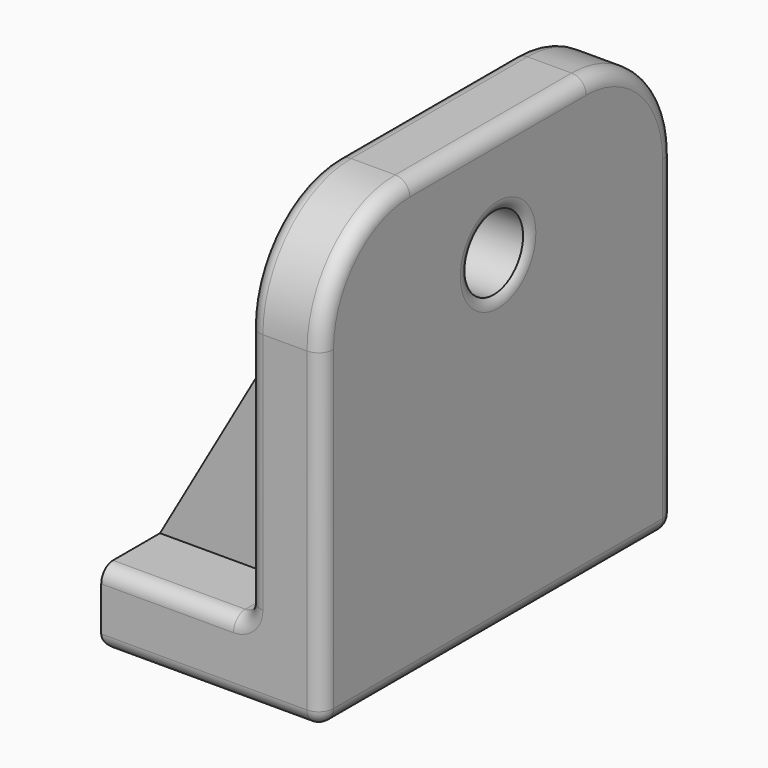
from build123d import *

# Parameters (mm, degrees)
F1_DEPTH  = 76.2
F2_R      = 12.7
F3_DEPTH  = 76.201
F5_DEPTH  = 25.401
F6_R      = 38.1
F7_R      = 38.1
F10_DEPTH = 6.35
F11_SIZE  = 1.524
F12_SIZE  = 1.524
F13_R     = 5.08


# Not quite as in the source:
# - a length typed as a fraction of an inch, garbled in the dataset ("3 / 203.2 mm" for 3/8 in), is restored
# - a pattern or mirror of a feature is missing from the dataset's text; its kind, count and spacing are read off the source's solid


with BuildPart() as f1:
    # F0 (on Front) → F1 (new body, symmetric)
    with BuildSketch(Plane.XZ):
        Polygon((-76.2, 0), (0, 0), (0, 152.4), (-25.4, 152.4), (-25.4, 25.4), (-76.2, 25.4), align=None)
    extrude(amount=F1_DEPTH, both=True)

    # F2 (on face) → F3 (cut, through all)
    with BuildSketch(Plane.YZ):
        with Locations((0, 114.3)):
            Circle(F2_R)
    extrude(amount=-F3_DEPTH, mode=Mode.SUBTRACT)

    # F4 (on face) → F5 (cut, through all)
    with BuildSketch(Plane.XY.offset(25.4)):
        with BuildLine():
            ThreePointArc((-63.5, -12.7), (-50.8, 0), (-63.5, 12.7))
            Line((-63.5, 12.7), (-76.2, 12.7))
            Line((-76.2, 12.7), (-76.2, -12.7))
            Line((-76.2, -12.7), (-63.5, -12.7))
        make_face()
    extrude(amount=-F5_DEPTH, mode=Mode.SUBTRACT)

    # F6
    f6_edges = [f1.edges().sort_by_distance(p)[0] for p in [
        (-12.7, 76.2, 152.4),
    ]]
    fillet(f6_edges, radius=F6_R)

    # F7
    f7_edges = [f1.edges().sort_by_distance(p)[0] for p in [
        (-12.7, -76.2, 152.4),
    ]]
    fillet(f7_edges, radius=F7_R)

    # F9 (on offset) → F10 (join, symmetric)
    with BuildSketch(Plane.XZ.offset(44.45)):
        Polygon((-76.2, 25.4), (-25.4, 25.4), (-25.4, 114.3), align=None)
    f10 = extrude(amount=F10_DEPTH, both=True)

    # F10_copies: F10 across plane
    add(f10.mirror(Plane.ZX))

    # F11
    f11_edges = [f1.edges().sort_by_distance(p)[0] for p in [
        (0, -12.7, 114.3),
        (-12.7, 12.7, 114.3),
        (-25.4, -12.7, 114.3),
    ]]
    chamfer(f11_edges, length=F11_SIZE)

    # F12
    f12_edges = [f1.edges().sort_by_distance(p)[0] for p in [
        (-25.4, -14.224, 114.3),
    ]]
    chamfer(f12_edges, length=F12_SIZE)

    # F13
    f13_edges = [f1.edges().sort_by_distance(p)[0] for p in [
        (-25.4, -15.748, 114.3),
        (-25.4, -65.040768, 141.240768),
        (-25.4, -76.2, 69.85),
        (-25.4, -63.5, 25.4),
        (-25.4, -50.8, 69.85),
        (-25.4, -44.45, 114.3),
        (-25.4, -38.1, 69.85),
        (-25.4, 0, 25.4),
        (-25.4, 38.1, 69.85),
        (-25.4, 44.45, 114.3),
        (-25.4, 50.8, 69.85),
        (-25.4, 63.5, 25.4),
        (-25.4, 76.2, 69.85),
        (-25.4, 65.040768, 141.240768),
        (-25.4, 0, 152.4),
        (-12.7, -38.1, 152.4),
        (-12.7, 38.1, 152.4),
        (0, 0, 152.4),
        (0, 65.040768, 141.240768),
        (-12.7, 76.2, 114.3),
        (0, -65.040768, 141.240768),
        (-12.7, -76.2, 114.3),
        (0, -14.224, 114.3),
        (0, -76.2, 57.15),
        (0, 76.2, 57.15),
        (0, 0, 0),
        (-76.2, 44.45, 0),
        (-69.85, 12.7, 0),
        (-50.8, 0, 0),
        (-69.85, -12.7, 0),
        (-76.2, -44.45, 0),
        (-38.1, -76.2, 0),
        (-38.1, 76.2, 0),
        (-50.8, -76.2, 25.4),
        (-50.8, 76.2, 25.4),
    ]]
    fillet(f13_edges, radius=F13_R)


solid = f1.part
